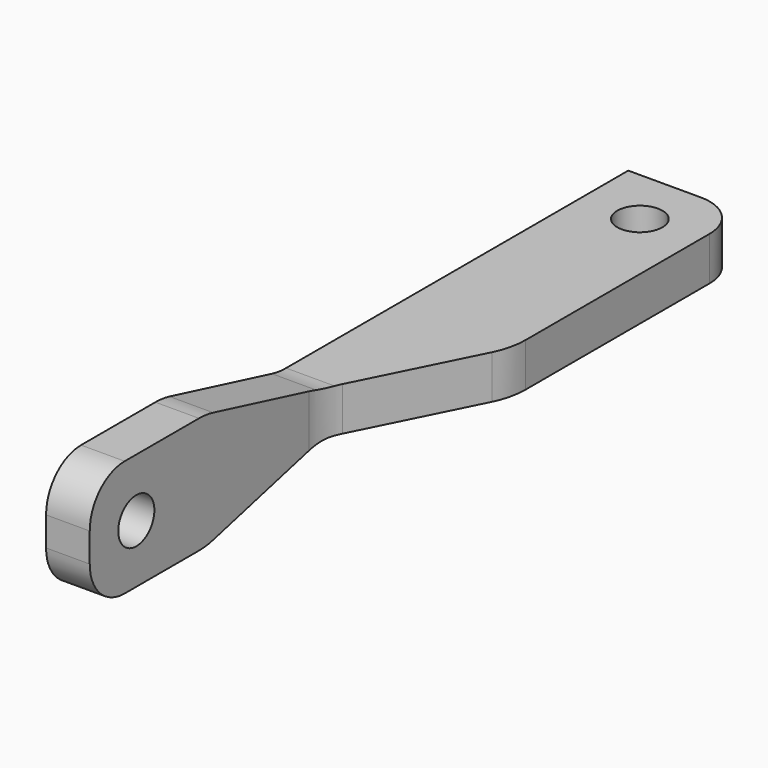
from build123d import *

# Parameters (mm, degrees)
F0_R     = 1.55
F0_W     = 30
F0_H     = 3
F1_DEPTH = 3
F2_W     = 30
F2_H     = 3
F3_DEPTH = 5
F4_R     = 1.55
F5_DEPTH = 3
F6_R     = 3
F7_F1_R  = 5
F7_F2_R  = 5
F7_F3_R  = 5
F7_F4_R  = 5
F7_F5_R  = 5
F7_F6_R  = 5


with BuildPart() as f1:
    # F0 (on Right) → F1 (new body)
    with BuildSketch(Plane.YZ):
        Polygon((-15, 4), (-25, 4), (-25, -4), (-15, -4), (-5, -1.5), (-5, 1.5), align=None)
        with Locations((-21, 0)):
            Circle(F0_R, mode=Mode.SUBTRACT)
        with Locations((10, 0)):
            Rectangle(F0_W, F0_H)
    extrude(amount=F1_DEPTH)

    # F2 (on face) → F3 (join)
    with BuildSketch(Plane.YZ.offset(3)):
        with Locations((10, 0)):
            Rectangle(F2_W, F2_H)
    extrude(amount=F3_DEPTH)

    # F4 (on face) → F5 (cut, through all)
    with BuildSketch(Plane(origin=(0, 0, -1.5), x_dir=(1, 0, 0), z_dir=(0, 0, -1))):
        Polygon((8, 5), (3, 5), (8, -5), align=None)
        with Locations((4, -21)):
            Circle(F4_R)
    extrude(amount=-F5_DEPTH, mode=Mode.SUBTRACT)

    # F6
    f6_edges = [f1.edges().sort_by_distance(p)[0] for p in [
        (1.5, -25, 4),
        (1.5, -25, -4),
        (8, 25, 0),
    ]]
    fillet(f6_edges, radius=F6_R)

    # F7: fillet of radius 5 on 6 edges, made by hand

    # F7_f1
    f7_f1_edges = [f1.edges().sort_by_distance(p)[0] for p in [
        (1.5, -15, 4),
    ]]
    fillet(f7_f1_edges, radius=F7_F1_R)

    # F7_f2
    f7_f2_edges = [f1.edges().sort_by_distance(p)[0] for p in [
        (1.5, -5, 1.5),
    ]]
    fillet(f7_f2_edges, radius=F7_F2_R)

    # F7_f3
    f7_f3_edges = [f1.edges().sort_by_distance(p)[0] for p in [
        (3, -5, 0.019016066),
    ]]
    fillet(f7_f3_edges, radius=F7_F3_R)

    # F7_f4
    f7_f4_edges = [f1.edges().sort_by_distance(p)[0] for p in [
        (1.5, -15, -4),
    ]]
    fillet(f7_f4_edges, radius=F7_F4_R)

    # F7_f5
    f7_f5_edges = [f1.edges().sort_by_distance(p)[0] for p in [
        (1.5706586412, -5, -1.5),
    ]]
    fillet(f7_f5_edges, radius=F7_F5_R)

    # F7_f6
    f7_f6_edges = [f1.edges().sort_by_distance(p)[0] for p in [
        (8, 5, 0),
    ]]
    fillet(f7_f6_edges, radius=F7_F6_R)


solid = f1.part
